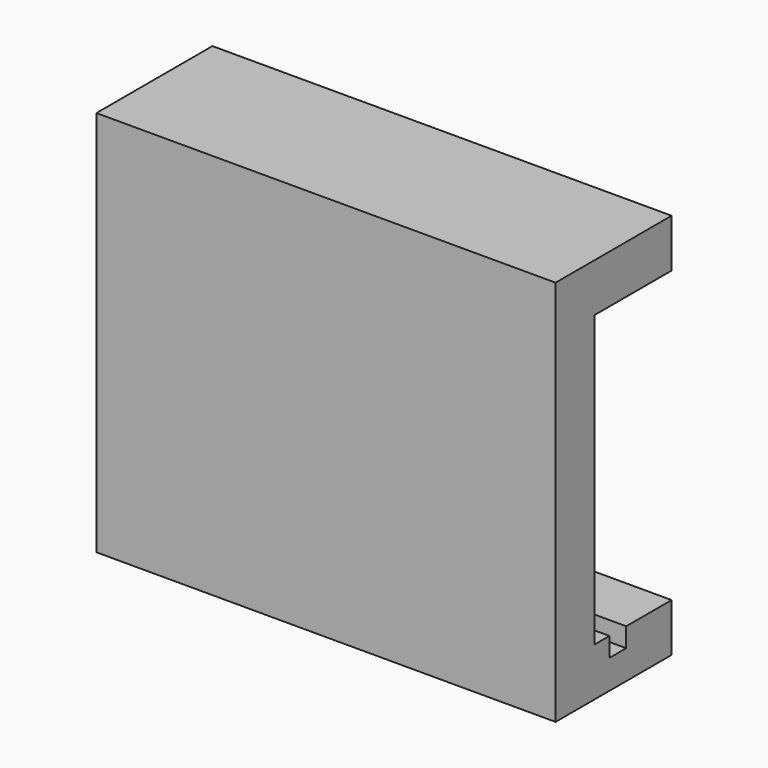
from build123d import *

# Parameters (mm, degrees)
F1_DEPTH = 203.2
F0_W     = 228.6
F0_H     = 10
F2_DEPTH = 25.4
F0_H_2   = 29.8
F0_H_3   = 11
F3_DEPTH = 15.24
F4_W     = 228.6
F4_H     = 50.8
F5_DEPTH = 25.4
F6_W     = 33.1639014184
F6_H     = 23.3497917652
F7_DEPTH = 25.4
F8_W     = 231.14
F8_H     = 60.0164352887
F9_DEPTH = 0.254


# Not quite as in the source:
# - a feature names something its author has since deleted; it is built from what else it names


with BuildPart() as f1:
    # F0 (on Top) → F1 (new body)
    with BuildSketch(Plane.XY):
        Polygon((-143.864646554, -49.5614223182), (97.435353446, -49.5614223182), (97.435353446, -24.1614223182), (-131.164646554, -24.1614223182), (-131.164646554, -14.1614223182), (-131.164646554, -3.1614223182), (-131.164646554, 26.6385776818), (-143.864646554, 26.6385776818), align=None)
    extrude(amount=F1_DEPTH)

    # F4 (on face) → F5 (join)
    with BuildSketch(Plane.XY.offset(203.2)):
        with Locations((-16.864646554, 1.2385776818)):
            Rectangle(F4_W, F4_H)
    extrude(amount=-F5_DEPTH)



with BuildPart() as f2:
    # F0 (on Top) → F2 (new body)
    with BuildSketch(Plane.XY):
        with Locations((-16.864646554, -19.1614223182)):
            Rectangle(F0_W, F0_H)
    extrude(amount=F2_DEPTH)


with BuildPart() as f2b:
    # F0 (on Top) → F2, piece 2 (new body)
    with BuildSketch(Plane.XY):
        with Locations((-16.864646554, 11.7385776818)):
            Rectangle(F0_W, F0_H_2)
    extrude(amount=F2_DEPTH)


with BuildPart() as f3:
    # F0 (on Top) → F3 (new body)
    with BuildSketch(Plane.XY):
        with Locations((-16.864646554, -8.6614223182)):
            Rectangle(F0_W, F0_H_3)
    extrude(amount=F3_DEPTH)


with BuildPart() as f1_1:
    add(f1.part)

    add(f2.part)  # F7 merges F2
    # F6 (on face) → F7 (join)
    with BuildSketch(Plane.YZ.offset(97.435353446)):
        with Locations((-32.979471609, 11.6748958826)):
            Rectangle(F6_W, F6_H)
    extrude(amount=-F7_DEPTH)


    add(f2b.part)  # F9 merges F2b

    add(f3.part)  # F9 merges F3
    # F8 (on face) → F9 (join)
    with BuildSketch(Plane(origin=(0, 0, 0), x_dir=(1, 0, 0), z_dir=(0, 0, -1))):
        with Locations((-18.134646554, 3.3696399626)):
            Rectangle(F8_W, F8_H)
    extrude(amount=-F9_DEPTH)


solid = f1_1.part
